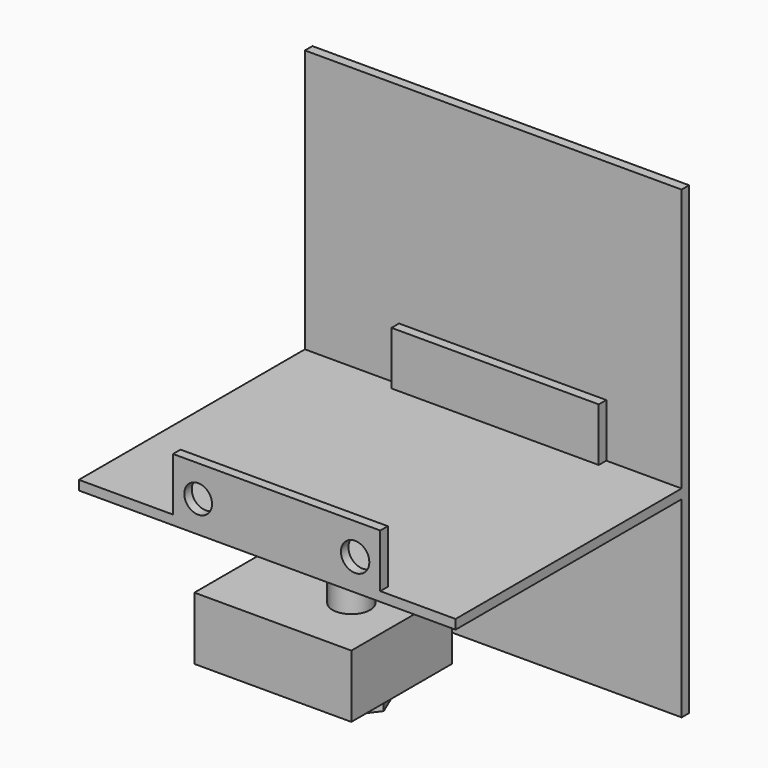
from build123d import *

# Parameters (mm, degrees)
F0_W      = 60
F0_H      = 74
F1_DEPTH  = 1.5
F2_W      = 33
F2_H      = 10
F3_DEPTH  = 1.5
F5_DEPTH  = 1.5
F6_W      = 33
F6_H      = 8.5
F6_H_2    = 1.5
F7_DEPTH  = 1.5
F8_R      = 2.2151606022
F8_R_2    = 2.2615912584
F9_DEPTH  = 2.5
F10_R     = 3
F11_DEPTH = 17
F12_W     = 25
F12_H     = 20
F12_R     = 3
F13_DEPTH = 10
F15_DEPTH = 3
F16_R     = 2.5
F17_DEPTH = 3
F18_SIZE2 = 2.99999
F18_SIZE  = 1.99999


# Not quite as in the source:
# - a fillet or chamfer is up to 0.001 mm smaller than in the source, because OpenCascade refuses the exact size


with BuildPart() as f1:
    # F0 (on Front) → F1 (new body)
    with BuildSketch(Plane.XZ):
        with Locations((-0.6031179801, 17)):
            Rectangle(F0_W, F0_H)
    extrude(amount=F1_DEPTH)

    # F2 (on face) → F3 (join)
    with BuildSketch(Plane.XZ.offset(1.5)):
        with Locations((0.8968820199, 15.5949131586)):
            Rectangle(F2_W, F2_H)
    extrude(amount=F3_DEPTH)

    # F4 (on face) → F5 (join)
    with BuildSketch(Plane(origin=(0, 0, 10.5949131586), x_dir=(1, 0, 0), z_dir=(0, 0, -1))):
        Polygon((-30.6031179801, 46.5), (-30.6031179801, 1.5), (-15.6031179801, 1.5), (-15.6031179801, 3), (17.3968820199, 3), (17.3968820199, 1.5), (29.3968820199, 1.5), (29.3968820199, 46.5), align=None)
    extrude(amount=-F5_DEPTH)

    # F6 (on face) → F7 (join)
    with BuildSketch(Plane.XZ.offset(46.5)):
        with Locations((0.8968820199, 16.3449131586)):
            Rectangle(F6_W, F6_H)
        with Locations((0.8968820199, 11.3449131586)):
            Rectangle(F6_W, F6_H_2)
    extrude(amount=-F7_DEPTH)

    # F8 (on face) → F9 (cut, symmetric)
    with BuildSketch(Plane.XZ.offset(46.5)):
        with Locations((-11.6031179801, 15.5949131586)):
            Circle(F8_R)
        with Locations((13.3968820199, 15.5949131586)):
            Circle(F8_R_2)
    extrude(amount=F9_DEPTH, both=True, mode=Mode.SUBTRACT)

    # F10 (on face) → F11 (join)
    with BuildSketch(Plane(origin=(0, 0, 10.5949131586), x_dir=(1, 0, 0), z_dir=(0, 0, -1))):
        with Locations((-5.6031179801, 23.5)):
            Circle(F10_R)
    extrude(amount=F11_DEPTH)

    # F12 (on face) → F13 (join)
    with BuildSketch(Plane(origin=(0, 0, -6.4050868414), x_dir=(1, 0, 0), z_dir=(0, 0, -1))):
        with Locations((-10.1031179801, 23.5)):
            Rectangle(F12_W, F12_H)
        with Locations((-5.6031179801, 23.5)):
            Circle(F12_R, mode=Mode.SUBTRACT)
        with Locations((-5.6031179801, 23.5)):
            Circle(F12_R)
    extrude(amount=F13_DEPTH)

    # F14 (on face) → F15 (join)
    with BuildSketch(Plane(origin=(0, 0, -16.4050868414), x_dir=(1, 0, 0), z_dir=(0, 0, -1))):
        Polygon((0.1261105875, 24.2136339076), (-3.3565287892, 28.8184744374), (-9.0857573568, 28.1048405298), (-11.3323465476, 22.7863660924), (-7.8497071709, 18.1815255626), (-2.1204786033, 18.8951594702), align=None)
    extrude(amount=F15_DEPTH)

    # F16 (on face) → F17 (join)
    with BuildSketch(Plane(origin=(0, 0, -19.4050868414), x_dir=(1, 0, 0), z_dir=(0, 0, -1))):
        with Locations((-5.6031179801, 23.5)):
            Circle(F16_R)
    extrude(amount=F17_DEPTH)

    # F18 (size 2 and 3 in the source; OpenCascade refuses exactly that, so slightly less here)
    f18_edges = [f1.edges().sort_by_distance(p)[0] for p in [
        (-8.103118, -23.5, -22.405087),
    ]]
    f18_side = f1.faces().sort_by_distance((-5.603118, -23.5, -22.405087))[0]
    chamfer(f18_edges, length=F18_SIZE, length2=F18_SIZE2, reference=f18_side)


solid = f1.part
